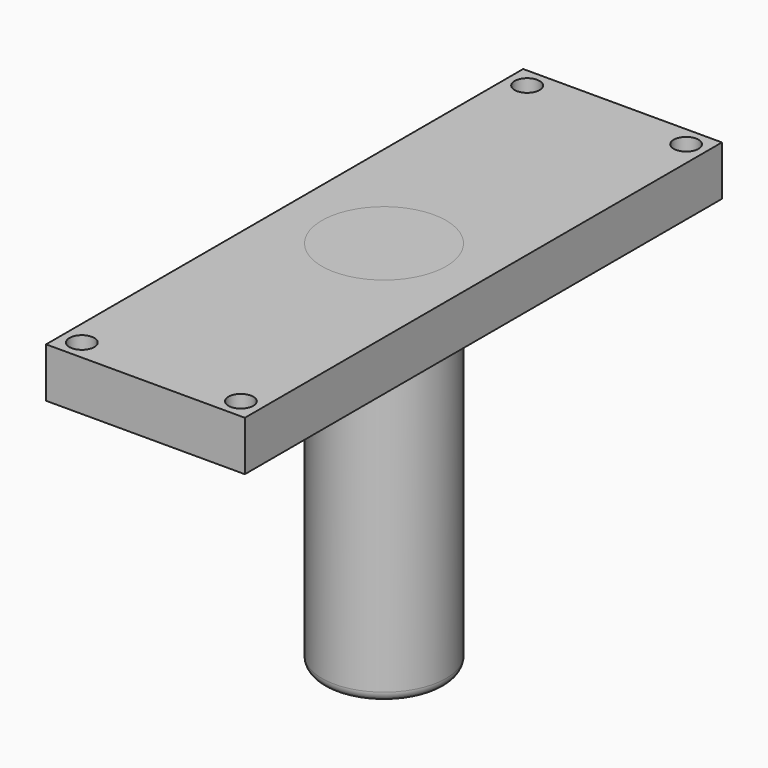
from build123d import *

# Parameters (mm, degrees)
F0_W     = 40
F0_H     = 120
F1_DEPTH = 10
F2_R     = 12.5
F3_DEPTH = 75
F2_R_2   = 2.5
F4_DEPTH = 25
F5_R     = 2
F6_R     = 3.8567448675
F7_DEPTH = 70


with BuildPart() as f1:
    # F0 (on Top) → F1 (new body)
    with BuildSketch(Plane.XY):
        Rectangle(F0_W, F0_H)
    extrude(amount=F1_DEPTH)

    # F2 (on face) → F4 (cut)
    with BuildSketch(Plane.XY.offset(10)):
        with Locations((-16, 56)):
            Circle(F2_R_2)
        with Locations((16, 56)):
            Circle(F2_R_2)
        with Locations((-16, -56)):
            Circle(F2_R_2)
        with Locations((16, -56)):
            Circle(F2_R_2)
        Circle(F2_R)
    extrude(amount=-F4_DEPTH, mode=Mode.SUBTRACT)


with BuildPart() as f3:
    # F2 (on face) → F3 (new body)
    with BuildSketch(Plane.XY.offset(10)):
        Circle(F2_R)
    extrude(amount=-F3_DEPTH)

    # F5
    f5_edges = [f3.edges().sort_by_distance(p)[0] for p in [
        (-12.5, 0, -65),
    ]]
    fillet(f5_edges, radius=F5_R)

    # F6 (on face) → F7 (cut)
    with BuildSketch(Plane(origin=(0, 0, -65), x_dir=(1, 0, 0), z_dir=(0, 0, -1))):
        Circle(F6_R)
    extrude(amount=-F7_DEPTH, mode=Mode.SUBTRACT)


solid = Compound([f1.part, f3.part])
